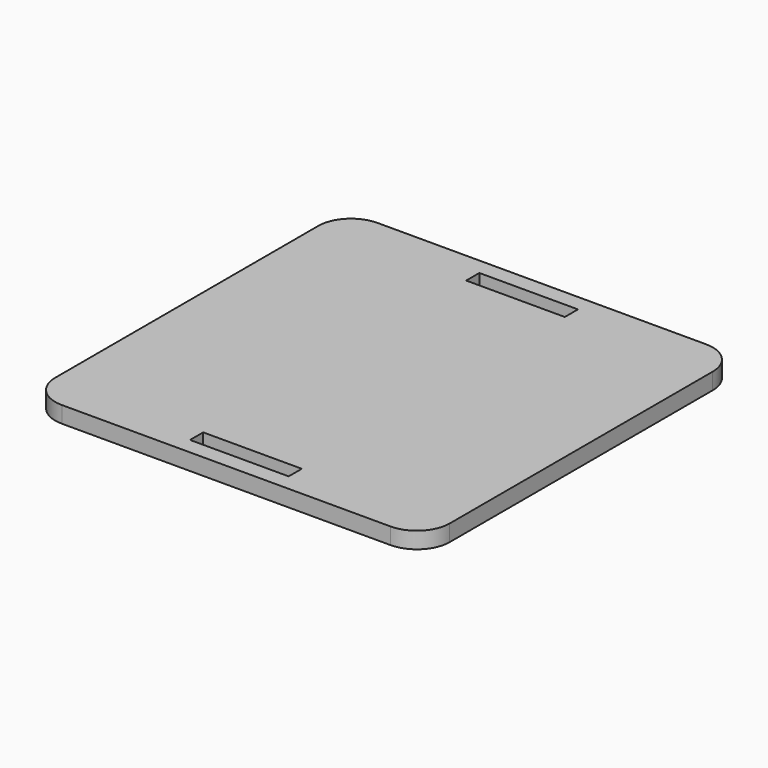
from build123d import *

# Parameters (mm, degrees)
F0_W     = 19.05
F0_H     = 3.175
F1_DEPTH = 3.175


# Not quite as in the source:
# - a length typed as a fraction of an inch, garbled in the dataset ("3 / 203.2 mm" for 3/8 in), is restored


with BuildPart() as f1:
    # F0 (on Top) → F1 (new body)
    with BuildSketch(Plane.XY):
        with BuildLine():
            Line((31.75, 38.1), (-31.75, 38.1))
            ThreePointArc((-31.75, 38.1), (-36.2401280605, 36.2401280605), (-38.1, 31.75))
            Line((-38.1, 31.75), (-38.1, -31.75))
            ThreePointArc((-38.1, -31.75), (-36.2401280605, -36.2401280605), (-31.75, -38.1))
            Line((-31.75, -38.1), (31.75, -38.1))
            ThreePointArc((31.75, -38.1), (36.2401280605, -36.2401280605), (38.1, -31.75))
            Line((38.1, -31.75), (38.1, 31.75))
            ThreePointArc((38.1, 31.75), (36.2401280605, 36.2401280605), (31.75, 38.1))
        make_face()
        with Locations((0, -33.3375)):
            Rectangle(F0_W, F0_H, mode=Mode.SUBTRACT)
        with Locations((0, 33.3375)):
            Rectangle(F0_W, F0_H, mode=Mode.SUBTRACT)
    extrude(amount=-F1_DEPTH)


solid = f1.part
